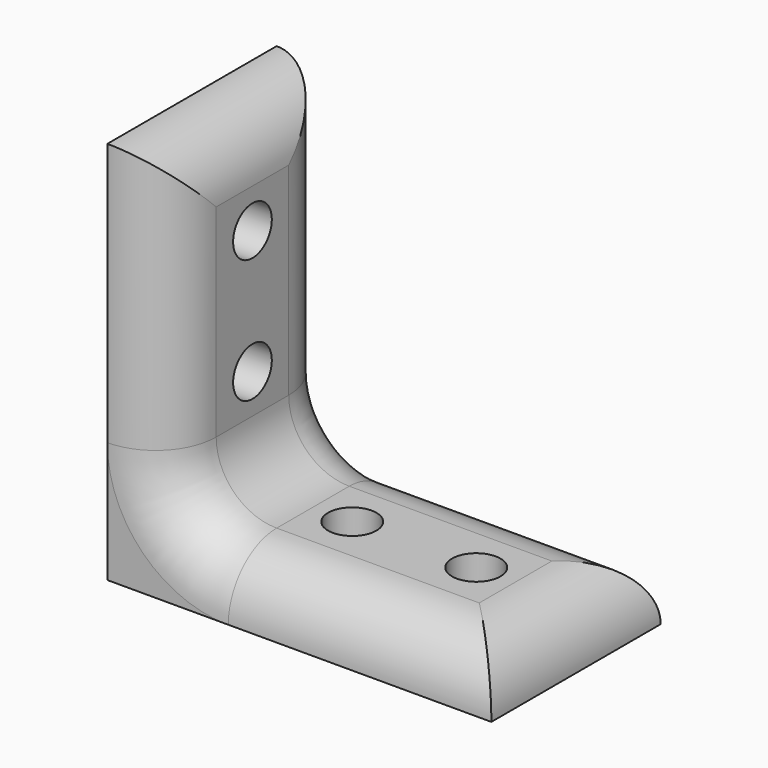
from build123d import *

# Parameters (mm, degrees)
F0_W     = 4
F0_H     = 14
F1_DEPTH = 25.4
F0_W_2   = 21.4
F0_R     = 1.6
F2_DEPTH = 4
F3_R     = 1.6
F4_DEPTH = 4
F5_F1_R  = 4
F5_F2_R  = 3.9999


# Not quite as in the source:
# - a fillet or chamfer is up to 0.001 mm smaller than in the source, because OpenCascade refuses the exact size


with BuildPart() as f1:
    # F0 (on Top) → F1 (new body)
    with BuildSketch(Plane.XY):
        with Locations((-8.6, 0)):
            Rectangle(F0_W, F0_H)
    extrude(amount=F1_DEPTH)

    # F0 (on Top) → F2 (join)
    with BuildSketch(Plane.XY):
        with Locations((4.1, 0)):
            Rectangle(F0_W_2, F0_H)
        Circle(F0_R, mode=Mode.SUBTRACT)
        with Locations((8.2, 0)):
            Circle(F0_R, mode=Mode.SUBTRACT)
    extrude(amount=F2_DEPTH)

    # F3 (on face) → F4 (cut, through all)
    with BuildSketch(Plane.YZ.offset(-6.6)):
        with Locations((0, 18.8)):
            Circle(F3_R)
        with Locations((0, 10.6)):
            Circle(F3_R)
    extrude(amount=-F4_DEPTH, mode=Mode.SUBTRACT)

    # F5: fillet of radius 4 on 5 edges, made by hand

    # F5_f1
    f5_f1_edges = [f1.edges().sort_by_distance(p)[0] for p in [
        (-6.6, 0, 4),
    ]]
    fillet(f5_f1_edges, radius=F5_F1_R)

    # F5_f2 (radius 4 in the source; OpenCascade refuses exactly that, so slightly less here)
    f5_f2_edges = [f1.edges().sort_by_distance(p)[0] for p in [
        (-6.6, 0, 25.4),
        (14.8, 0, 4),
        (-6.6, 7, 16.7),
        (6.1, -7, 4),
        (-5.4284271247, -7, 5.1715728753),
        (-5.4284271247, 7, 5.1715728753),
    ]]
    fillet(f5_f2_edges, radius=F5_F2_R)


solid = f1.part
